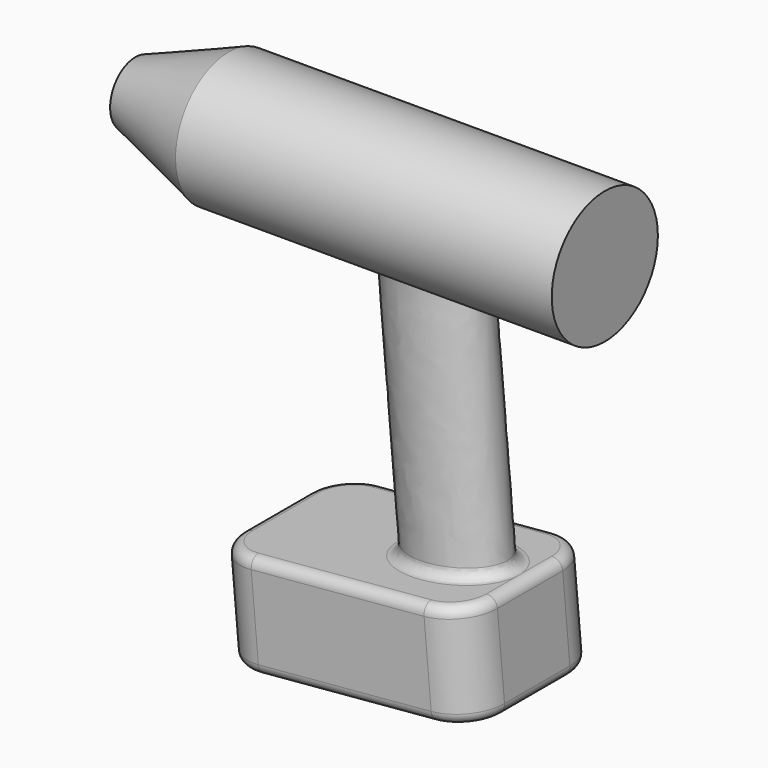
from build123d import *

# Parameters (mm, degrees)
F0_R          = 32.5
F1_DEPTH      = 85
F1_DEPTH_BACK = 145
F5_DEPTH      = 150
F7_W          = 125
F7_H          = 80
F8_DEPTH      = 50
F11_R         = 20
F12_R         = 4.99999


# Not quite as in the source:
# - a fillet or chamfer is up to 0.001 mm smaller than in the source, because OpenCascade refuses the exact size


with BuildPart() as f1:
    # F0 (on Right) → F1 (new body, two sides)
    with BuildSketch(Plane.YZ) as f1_sk:
        Circle(F0_R)
    extrude(amount=F1_DEPTH)
    extrude(f1_sk.sketch, amount=-F1_DEPTH_BACK)

    # F4 (on line) → F5 (join)
    with BuildSketch(Plane(origin=(0, 0, 0), x_dir=(0.9961946981, 0, 0.0871557427), z_dir=(0.0871557427, 0, -0.9961946981))):
        with BuildLine():
            add(Edge.make_bspline(
                [(25, 0), (25, 30.3108891325), (-12.5, 15.1554445662), (-50, 0), (-12.5, -15.1554445662), (25, -30.3108891325), (25, 0)],
                knots=[0, 0, 0, 2.0943951024, 2.0943951024, 4.1887902048, 4.1887902048, 6.2831853072, 6.2831853072, 6.2831853072], degree=2, weights=[1, 0.5, 1, 0.5, 1, 0.5, 1]))
        make_face()
    extrude(amount=F5_DEPTH)

    # F7 (on offset) → F8 (join)
    with BuildSketch(Plane(origin=(13.0733614121, 0, -149.4292047138), x_dir=(0.9961946981, 0, 0.0871557427), z_dir=(0.0871557427, 0, -0.9961946981))):
        with Locations((-27.5, 0)):
            Rectangle(F7_W, F7_H)
    extrude(amount=F8_DEPTH)

    # F9 (on Front) → F10 (revolve, cut)
    with BuildSketch(Plane.XZ):
        Polygon((-145, 32.5), (-145, 15.4653014615), (-99.2988270521, 32.5), align=None)
    revolve(axis=Axis((-67.4336478114, 0, 0), (1, 0, 0)), mode=Mode.SUBTRACT)

    # F11
    f11_edges = [f1.edges().sort_by_distance(p)[0] for p in [
        (-74.405268, 40, -182.178089),
        (-74.405268, -40, -182.178089),
        (50.119069, -40, -171.283621),
        (50.119069, 40, -171.283621),
    ]]
    fillet(f11_edges, radius=F11_R)

    # F12 (radius 5 in the source; OpenCascade refuses exactly that, so slightly less here)
    f12_edges = [f1.edges().sort_by_distance(p)[0] for p in [
        (-11.831506, 0, -151.608098),
        (47.940176, 0, -146.378754),
        (42.104602, 34.142136, -146.8893),
        (42.104602, -34.142136, -146.8893),
        (-14.321993, 40, -151.825988),
        (-14.321993, -40, -151.825988),
        (-70.748588, 34.142136, -156.762675),
        (-70.748588, -34.142136, -156.762675),
        (-76.584161, 0, -157.273222),
        (52.297963, 0, -196.188489),
        (46.46239, 34.142136, -196.699035),
        (46.46239, -34.142136, -196.699035),
        (-9.964206, 40, -201.635723),
        (-9.964206, -40, -201.635723),
        (-66.390801, 34.142136, -206.57241),
        (-66.390801, -34.142136, -206.57241),
        (-72.226374, 0, -207.082956),
    ]]
    fillet(f12_edges, radius=F12_R)


solid = f1.part
